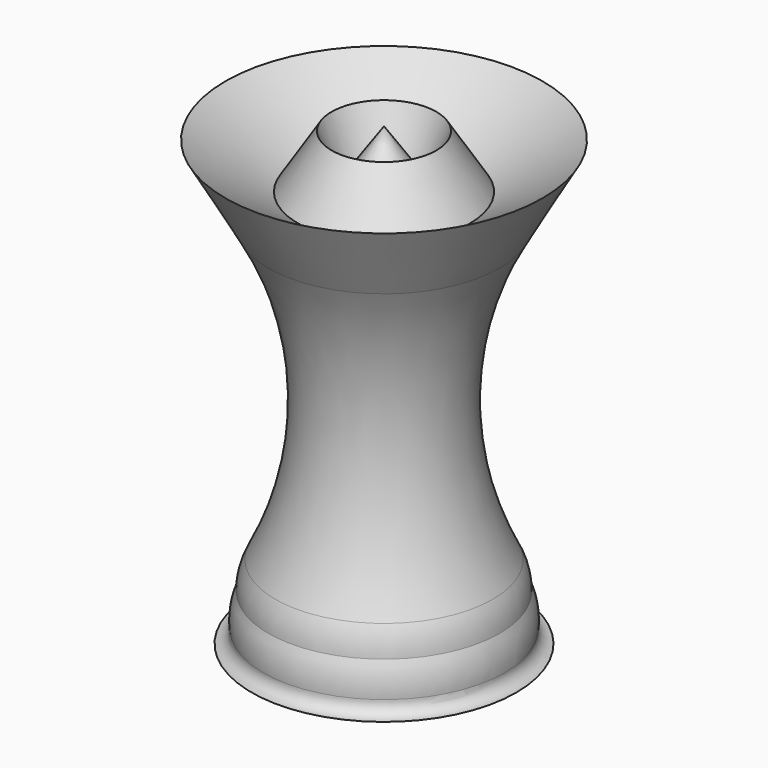
from build123d import *


# Not quite as in the source:
# - a fillet or chamfer that OpenCascade refuses, or shapes differently, is made with other operations: its cross-section is extruded or revolved along the edge and cut away or added


with BuildPart() as f1:
    # F0 (on Front) → F1 (revolve)
    with BuildSketch(Plane.XZ):
        with BuildLine():
            Line((0, 7.1883308701), (0, -30.2243120968))
            Line((0, -30.2243120968), (10.8706858009, -30.2243120968))
            ThreePointArc((10.8706858009, -30.2243120968), (9.889180772, -29.2428070679), (10.8706858009, -28.261302039))
            Line((10.8706858009, -28.261302039), (9.4850324094, -26.413762942))
            Line((9.4850324094, -26.413762942), (9.4850324094, -25.1435805112))
            ThreePointArc((9.4850324094, -25.1435805112), (6.1587538552, -12.5717902556), (9.4850324094, 0))
            Line((9.4850324094, 0), (13.0181515325, 6.2093746912))
            Line((13.0181515325, 6.2093746912), (7.0601375774, 2.4540154263))
            Line((7.0601375774, 2.4540154263), (4.3007276076, 6.8319196288))
            Line((4.3007276076, 6.8319196288), (2.7877071407, 3.1468416564))
            Line((2.7877071407, 3.1468416564), (0, 7.1883308701))
        make_face()
    revolve(axis=Axis((0, 0, -11.5179906134), (0, 0, -1)))

    # F2: fillet of radius 5.08 on 3 edges, made by hand

    # F2_s1 → F2_t2 (revolve, cut)
    with BuildSketch(Plane.XZ):
        with BuildLine():
            ThreePointArc((9.8965199445, -29.1230030365), (9.8769062732, -27.7401129903), (9.4850324094, -26.413762942))
            Line((9.4850324094, -26.413762942), (9.577642948, -26.3719795942))
            ThreePointArc((9.577642948, -26.3719795942), (10.2591391248, -27.2765725167), (10.9519658206, -28.2003420652))
            Line((10.9519658206, -28.2003420652), (10.8706858009, -28.362902039))
            ThreePointArc((10.8706858009, -28.362902039), (10.2877069025, -28.5837407102), (9.9973602337, -29.1354044906))
            Line((9.9973602337, -29.1354044906), (9.8965199445, -29.1230030365))
        make_face()
    revolve(axis=Axis((0, 0, -28.261302039), (0, 0, -1)), mode=Mode.SUBTRACT)

    # F2_s3 → F2_t4 (revolve, cut)
    with BuildSketch(Plane.XZ):
        with BuildLine():
            ThreePointArc((9.4850324094, -26.413762942), (9.3435632486, -25.2320724327), (8.9310390894, -24.1157258013))
            Line((8.9310390894, -24.1157258013), (9.0215590688, -24.0695880366))
            ThreePointArc((9.0215590688, -24.0695880366), (9.2915699789, -24.584629862), (9.5733382381, -25.0933347091))
            Line((9.5733382381, -25.0933347091), (9.5866324094, -25.1435805112))
            Line((9.5866324094, -25.1435805112), (9.5866322552, -26.4135859201))
            Line((9.5866322552, -26.4135859201), (9.4850324094, -26.413762942))
        make_face()
    revolve(axis=Axis((0, 0, -25.1435805112), (0, 0, -1)), mode=Mode.SUBTRACT)


solid = f1.part
